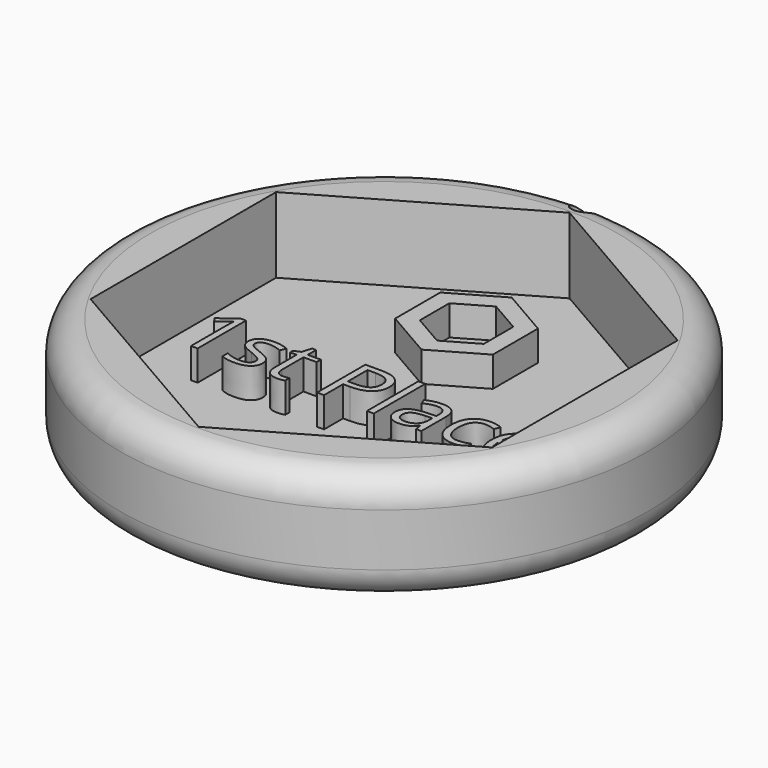
from build123d import *

# Parameters (mm, degrees)
F0_R         = 44.45
F1_DEPTH     = 19.05
F3_DEPTH     = 12.7
F4_R         = 1.8776509991
F5_DEPTH     = 40.513
F6_TEXT_SIZE = 14.2515675786
F7_DEPTH     = 5.08
F9_DEPTH     = 5.08
F11_DEPTH    = 5.08


# Not quite as in the source:
# - a fillet or chamfer that OpenCascade refuses, or shapes differently, is made with other operations: its cross-section is extruded or revolved along the edge and cut away or added
# - Text() gives the source's letters only with a copy of the font that has no kerning and outlines rounded to 1/6400 em; it was checked with that copy


with BuildPart() as f1:
    # F0 (on Top) → F1 (new body)
    with BuildSketch(Plane.XY):
        Circle(F0_R)
    extrude(amount=F1_DEPTH)

    # F2 (on face) → F3 (cut)
    with BuildSketch(Plane.XY.offset(19.05)):
        Polygon((33.8113345206, -19.5209830871), (33.8113345206, 19.5209830871), (0, 39.0419661742), (-33.8113345206, 19.5209830871), (-33.8113345206, -19.5209830871), (0, -39.0419661742), align=None)
    extrude(amount=-F3_DEPTH, mode=Mode.SUBTRACT)

    # F4 (on face) → F5 (cut)
    with BuildSketch(Plane.XY.offset(19.05)):
        with Locations((-0.0029054779, 41.8906919658)):
            Circle(F4_R)
    extrude(amount=-F5_DEPTH, mode=Mode.SUBTRACT)

    # F6 (on face) → F7 (join)
    with BuildSketch(Plane.XY.offset(6.35)):
        with Locations((-28.1600299586, -10.2611286566)):
            Text('1st Place', F6_TEXT_SIZE, font='Open Sans', text_align=(TextAlign.LEFT, TextAlign.BOTTOM))
    extrude(amount=F7_DEPTH)

    # F8 (on face) → F9 (join)
    with BuildSketch(Plane.XY.offset(6.35)):
        Polygon((8.2243764773, 12.614230005), (8.2243764773, 22.1109219511), (0, 26.8592679242), (-8.2243764773, 22.1109219511), (-8.2243764773, 12.614230005), (0, 7.8658840319), align=None)
    extrude(amount=F9_DEPTH)

    # F10 (on face) → F11 (cut)
    with BuildSketch(Plane.XY.offset(11.43)):
        Polygon((5.3813825361, 14.2556333222), (5.3813825361, 20.4695186339), (0, 23.5764612897), (-5.3813825361, 20.4695186339), (-5.3813825361, 14.2556333222), (0, 11.1486906663), align=None)
    extrude(amount=-F11_DEPTH, mode=Mode.SUBTRACT)

    # F12: fillet of radius 5.08 on 2 edges, made by hand

    # F12_s1 → F12_t2 (revolve, cut)
    with BuildSketch(Plane.XZ):
        with BuildLine():
            ThreePointArc((44.45, 13.97), (42.9621024484, 17.5621024484), (39.37, 19.05))
            Line((39.37, 19.05), (44.45, 19.05))
            Line((44.45, 19.05), (44.45, 13.97))
        make_face()
    revolve(axis=Axis((0, 0, 19.05), (0, 0, 1)), mode=Mode.SUBTRACT)

    # F12_s3 → F12_t4 (revolve, cut)
    with BuildSketch(Plane.XZ):
        with BuildLine():
            ThreePointArc((44.45, 5.08), (42.9621024484, 1.4878975516), (39.37, 0))
            Line((39.37, 0), (44.45, 0))
            Line((44.45, 0), (44.45, 5.08))
        make_face()
    revolve(axis=Axis((0, 0, 0), (0, 0, 1)), mode=Mode.SUBTRACT)


solid = f1.part
